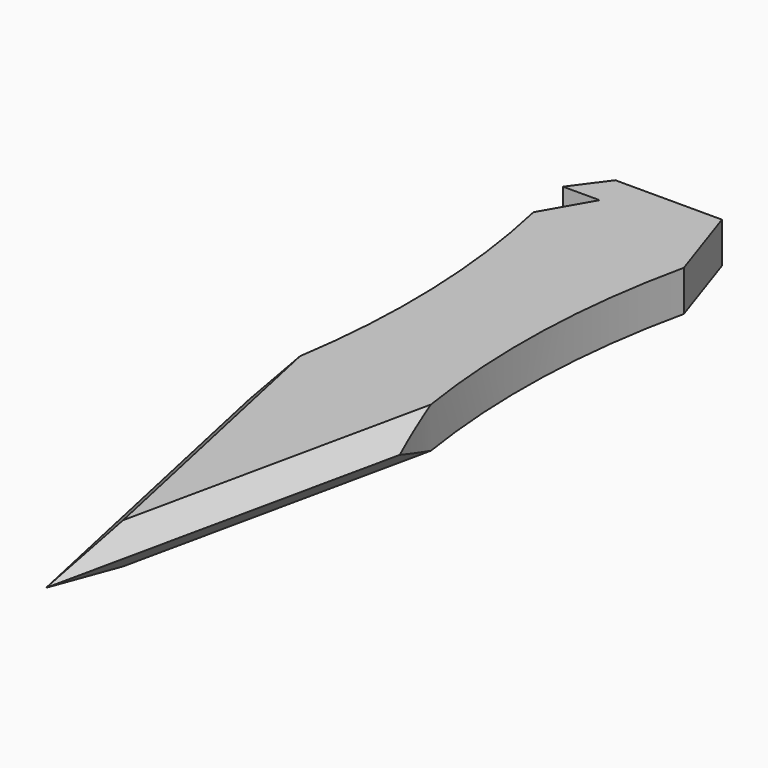
from build123d import *

# Parameters (mm, degrees)
F1_DEPTH = 6.35
F3_DEPTH = 25.4
F5_DEPTH = 6.35
F6_SIZE  = 3.17499


# Not quite as in the source:
# - a fillet or chamfer is up to 0.001 mm smaller than in the source, because OpenCascade refuses the exact size


with BuildPart() as f1:
    # F0 (on Top) → F1 (new body)
    with BuildSketch(Plane.XY):
        Polygon((-21.1028610796, 36.5512275749), (-11.7370359251, 20.3291425525), (0, 29.516665265), (11.7370359251, 20.3291425525), (33.4666037048, 57.9658579735), (26.5181194991, 63.6764243245), (35.1014384706, 60.7974748498), (47.9729409095, 83.0915710438), (43.2239025831, 86.8056491017), (49.1863254635, 85.1932147405), (60.325, 104.4859649666), (44.45, 109.9852262806), (0, 63.5), (-44.45, 109.9852262806), (-60.325, 104.4859649666), (-49.1863254635, 85.1932147405), (-43.2239025831, 86.8056491017), (-47.9729409095, 83.0915710438), (-35.1014384706, 60.7974748498), (-26.5181194991, 63.6764243245), (-33.4666037048, 57.9658579735), align=None)
    extrude(amount=F1_DEPTH)

    # F2 (on face) → F3 (cut)
    with BuildSketch(Plane(origin=(0, 0, 0), x_dir=(1, 0, 0), z_dir=(0, 0, -1))):
        with BuildLine():
            ThreePointArc((-11.7370359251, -75.7744380392), (-8.6743378245, -48.0517902958), (-11.7370359251, -20.3291425525))
            Line((-11.7370359251, -20.3291425525), (-33.4666037048, -57.9658579735))
            Line((-33.4666037048, -57.9658579735), (-26.5181194991, -63.6764243245))
            Line((-26.5181194991, -63.6764243245), (-35.1014384706, -60.7974748498))
            Line((-35.1014384706, -60.7974748498), (-47.9729409095, -83.0915710438))
            Line((-47.9729409095, -83.0915710438), (-43.2239025831, -86.8056491017))
            Line((-43.2239025831, -86.8056491017), (-49.1863254635, -85.1932147405))
            Line((-49.1863254635, -85.1932147405), (-60.325, -104.4859649666))
            Line((-60.325, -104.4859649666), (-44.45, -109.9852262806))
            Line((-44.45, -109.9852262806), (-11.7370359251, -75.7744380392))
        make_face()
        with BuildLine():
            Line((33.4666037048, -57.9658579735), (11.7370359251, -20.3291425525))
            ThreePointArc((11.7370359251, -20.3291425525), (8.6743378245, -48.0517902958), (11.7370359251, -75.7744380392))
            Line((11.7370359251, -75.7744380392), (44.45, -109.9852262806))
            Line((44.45, -109.9852262806), (60.325, -104.4859649666))
            Line((60.325, -104.4859649666), (49.1863254635, -85.1932147405))
            Line((49.1863254635, -85.1932147405), (43.2239025831, -86.8056491017))
            Line((43.2239025831, -86.8056491017), (47.9729409095, -83.0915710438))
            Line((47.9729409095, -83.0915710438), (35.1014384706, -60.7974748498))
            Line((35.1014384706, -60.7974748498), (26.5181194991, -63.6764243245))
            Line((26.5181194991, -63.6764243245), (33.4666037048, -57.9658579735))
        make_face()
    extrude(amount=-F3_DEPTH, mode=Mode.SUBTRACT)

    # F4 (on face) → F5 (join)
    with BuildSketch(Plane.XY.offset(6.35)):
        Polygon((-7.4254795909, 83.2857191563), (-11.7370359251, 75.7744380392), (0, 63.5), (11.7370359251, 75.7744380392), (7.4199811484, 88.5948985815), (-9.2232923578, 88.5948985815), (-13.126935586, 83.2857191563), align=None)
        Polygon((0, 29.516665265), (-11.7370359251, 20.3291425525), (0, -33.983334735), (11.7370359251, 20.3291425525), align=None)
    extrude(amount=-F5_DEPTH)

    # F6 (size 3.175 in the source; OpenCascade refuses exactly that, so slightly less here)
    f6_edges = [f1.edges().sort_by_distance(p)[0] for p in [
        (5.868518, -6.827096, 6.35),
        (-5.868518, -6.827096, 6.35),
        (5.868518, -6.827096, 0),
        (-5.868518, -6.827096, 0),
    ]]
    chamfer(f6_edges, length=F6_SIZE)


solid = f1.part
